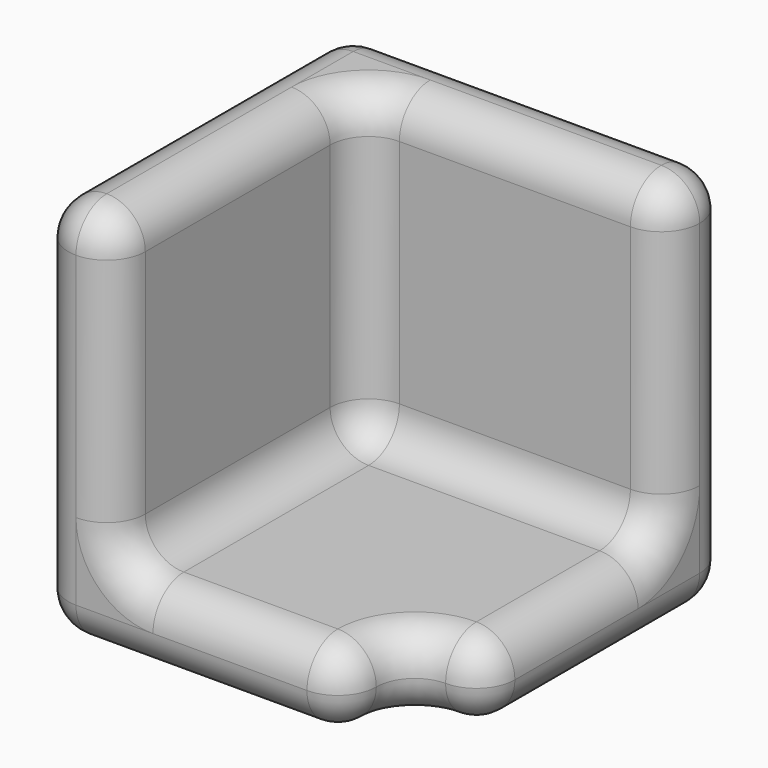
from build123d import *

# Parameters (mm, degrees)
F0_W     = 63.5
F0_H     = 63.5
F1_DEPTH = 63.5
F2_W     = 50.8
F2_H     = 50.8
F3_DEPTH = 50.8
F4_W     = 12.7
F4_H     = 12.7
F5_DEPTH = 12.7
F6_R     = 6.34999


# Not quite as in the source:
# - a fillet or chamfer is up to 0.001 mm smaller than in the source, because OpenCascade refuses the exact size


with BuildPart() as f1:
    # F0 (on Front) → F1 (new body)
    with BuildSketch(Plane.XZ):
        with Locations((31.75, -31.75)):
            Rectangle(F0_W, F0_H)
    extrude(amount=F1_DEPTH)

    # F2 (on face) → F3 (cut)
    with BuildSketch(Plane.XY):
        with Locations((38.1, -38.1)):
            Rectangle(F2_W, F2_H)
    extrude(amount=-F3_DEPTH, mode=Mode.SUBTRACT)

    # F4 (on face) → F5 (cut)
    with BuildSketch(Plane.XY.offset(-50.8)):
        with Locations((57.15, -57.15)):
            Rectangle(F4_W, F4_H)
    extrude(amount=-F5_DEPTH, mode=Mode.SUBTRACT)

    # F6 (radius 6.35 in the source; OpenCascade refuses exactly that, so slightly less here)
    f6_edges = [f1.edges().sort_by_distance(p)[0] for p in [
        (31.75, 0, 0),
        (0, -31.75, 0),
        (6.35, -63.5, 0),
        (12.7, -38.1, 0),
        (38.1, -12.7, 0),
        (63.5, -6.35, 0),
        (63.5, -50.8, -57.15),
        (50.8, -50.8, -57.15),
        (57.15, -50.8, -50.8),
        (57.15, -50.8, -63.5),
        (38.1, -12.7, -50.8),
        (63.5, -31.75, -50.8),
        (50.8, -57.15, -50.8),
        (31.75, -63.5, -50.8),
        (12.7, -38.1, -50.8),
        (63.5, 0, -31.75),
        (63.5, -12.7, -25.4),
        (63.5, -25.4, -63.5),
        (12.7, -63.5, -25.4),
        (50.8, -63.5, -57.15),
        (25.4, -63.5, -63.5),
        (0, -63.5, -31.75),
        (50.8, -57.15, -63.5),
        (31.75, 0, -63.5),
        (0, -31.75, -63.5),
        (12.7, -12.7, -25.4),
        (0, 0, -31.75),
    ]]
    fillet(f6_edges, radius=F6_R)


solid = f1.part
